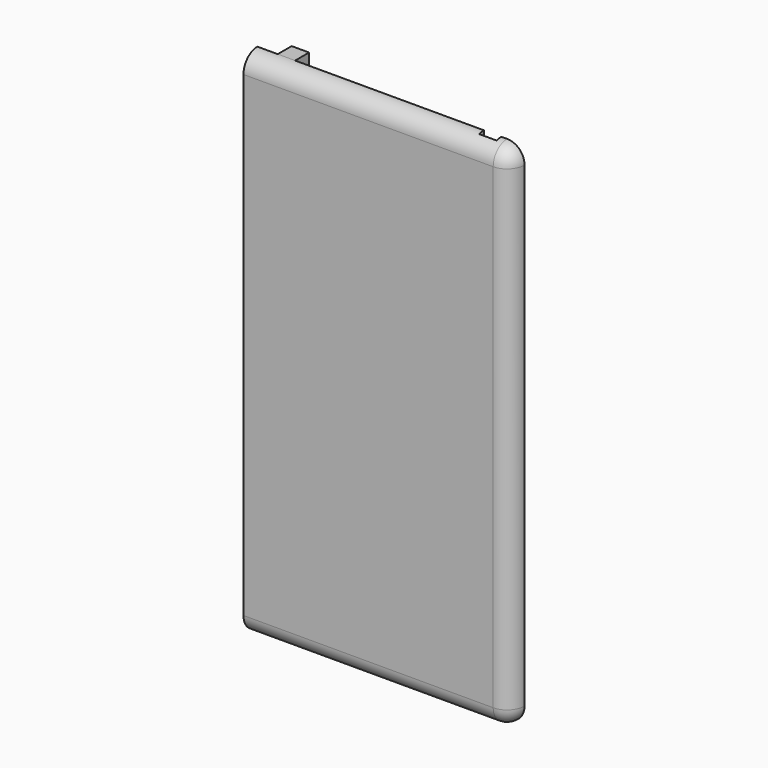
from build123d import *

# Parameters (mm, degrees)
F0_W         = 292.1
F0_H         = 558.8
F1_DEPTH     = 19.05
F3_W         = 19.05
F3_H         = 558.8
F4_DEPTH     = 6.35
F5_T1_DEPTH  = 320.675
F5_T3_DEPTH  = 520.7
F5_T5_DEPTH  = 47.625
F5_S9_W      = 19.05
F5_S9_H      = 19.05
F5_T10_DEPTH = 19.05
F5_S15_W     = 19.05
F5_S15_H     = 19.05
F5_T16_DEPTH = 19.05
F6_W         = 19.05
F6_H         = 558.8
F7_DEPTH     = 19.05


# Not quite as in the source:
# - a fillet or chamfer that OpenCascade refuses, or shapes differently, is made with other operations: its cross-section is extruded or revolved along the edge and cut away or added


with BuildPart() as f1:
    # F0 (on Front) → F1 (new body)
    with BuildSketch(Plane.XZ):
        Rectangle(F0_W, F0_H)
    extrude(amount=-F1_DEPTH)

    # F3 (on face) → F4 (cut)
    with BuildSketch(Plane(origin=(0, 19.05, 0), x_dir=(-1, 0, 0), z_dir=(0, 1, 0))):
        with Locations((-111.125, 0)):
            Rectangle(F3_W, F3_H)
    extrude(amount=-F4_DEPTH, mode=Mode.SUBTRACT)

    # F5: fillet of radius 19.05 on 5 edges, made by hand

    # F5_s2 → F5_t1 (cut)
    with BuildSketch(Plane.YZ.offset(-193.675)):
        with BuildLine():
            ThreePointArc((19.05, -279.4), (5.5796158184, -273.8203841816), (0, -260.35))
            Line((0, -260.35), (0, -279.4))
            Line((0, -279.4), (19.05, -279.4))
        make_face()
        with BuildLine():
            ThreePointArc((19.05, 279.4), (5.5796158184, 273.8203841816), (0, 260.35))
            Line((0, 260.35), (0, 279.4))
            Line((0, 279.4), (19.05, 279.4))
        make_face()
    extrude(amount=F5_T1_DEPTH, mode=Mode.SUBTRACT)

    # F5_s4 → F5_t3 (cut)
    with BuildSketch(Plane.XY.offset(-260.35)):
        with BuildLine():
            ThreePointArc((127, 0), (140.4703841816, 5.5796158184), (146.05, 19.05))
            Line((146.05, 19.05), (146.05, 0))
            Line((146.05, 0), (127, 0))
        make_face()
    extrude(amount=F5_T3_DEPTH, mode=Mode.SUBTRACT)

    # F5_s6 → F5_t5 (cut)
    with BuildSketch(Plane.XZ.offset(-66.675)):
        with BuildLine():
            ThreePointArc((127, -279.4), (140.4703841816, -273.8203841816), (146.05, -260.35))
            Line((146.05, -260.35), (146.05, -279.4))
            Line((146.05, -279.4), (127, -279.4))
        make_face()
        with BuildLine():
            ThreePointArc((127, 279.4), (140.4703841816, 273.8203841816), (146.05, 260.35))
            Line((146.05, 260.35), (146.05, 279.4))
            Line((146.05, 279.4), (127, 279.4))
        make_face()
    extrude(amount=F5_T5_DEPTH, mode=Mode.SUBTRACT)


with BuildPart() as f5_tool8:
    # F5_s9 → F5_t10 (new body)
    with BuildSketch(Plane.YZ.offset(127)):
        with Locations((9.525, -269.875)):
            Rectangle(F5_S9_W, F5_S9_H)
    extrude(amount=F5_T10_DEPTH)

    # F5_s11 → F5_t12 (revolve, cut)
    with BuildSketch(Plane(origin=(127, 19.05, -260.35), x_dir=(0, 0.7071067812, 0.7071067812), z_dir=(0, 0.7071067812, -0.7071067812))):
        with BuildLine():
            ThreePointArc((0, -19.05), (19.05, 0), (0, 19.05))
            Line((0, 19.05), (0, -19.05))
        make_face()
    revolve(axis=Axis((127, 19.05, -260.35), (1, 0, 0)), mode=Mode.SUBTRACT)


with BuildPart() as f1_1:
    add(f1.part)

    # F5_t7: cut F5_tool8
    add(f5_tool8.part, mode=Mode.SUBTRACT)


with BuildPart() as f5_tool14:
    # F5_s15 → F5_t16 (new body)
    with BuildSketch(Plane.YZ.offset(127)):
        with Locations((9.525, 269.875)):
            Rectangle(F5_S15_W, F5_S15_H)
    extrude(amount=F5_T16_DEPTH)

    # F5_s17 → F5_t18 (revolve, cut)
    with BuildSketch(Plane(origin=(127, 19.05, 260.35), x_dir=(0, 0.7071067812, -0.7071067812), z_dir=(0, -0.7071067812, -0.7071067812))):
        with BuildLine():
            ThreePointArc((0, -19.05), (19.05, 0), (0, 19.05))
            Line((0, 19.05), (0, -19.05))
        make_face()
    revolve(axis=Axis((127, 19.05, 260.35), (1, 0, 0)), mode=Mode.SUBTRACT)


with BuildPart() as f1_2:
    add(f1_1.part)

    # F5_t13: cut F5_tool14
    add(f5_tool14.part, mode=Mode.SUBTRACT)

    # F6 (on face) → F7 (join)
    with BuildSketch(Plane(origin=(0, 19.05, 0), x_dir=(-1, 0, 0), z_dir=(0, 1, 0))):
        with Locations((114.3, 0)):
            Rectangle(F6_W, F6_H)
    extrude(amount=F7_DEPTH)


solid = f1_2.part
